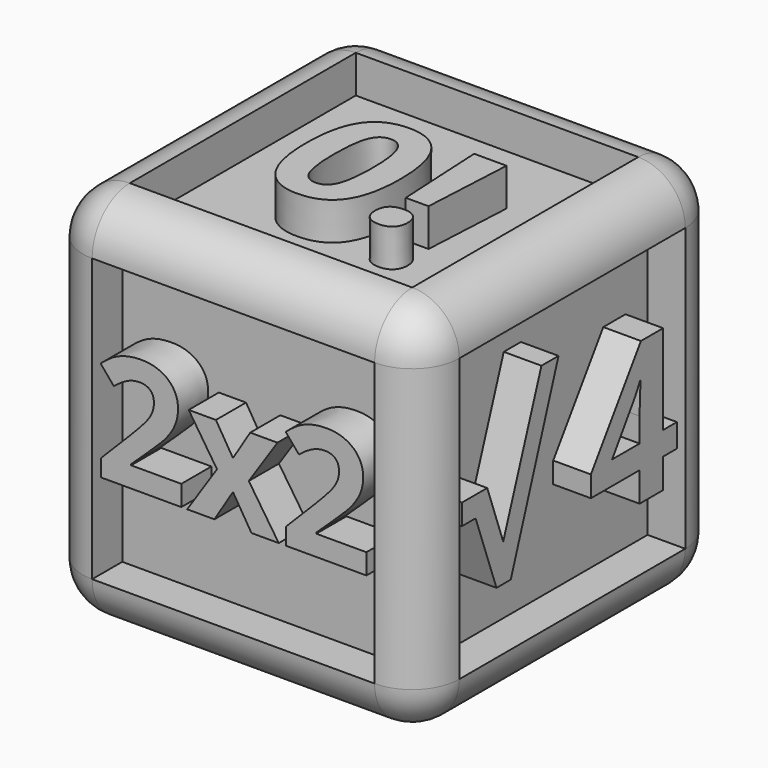
from build123d import *

# Parameters (mm, degrees)
F0_W          = 40
F0_H          = 40
F1_DEPTH      = 40
F2_R          = 5
F3_DEPTH      = 4
F4_DEPTH      = 4
F5_DEPTH      = 4
F6_DEPTH      = 4
F7_DEPTH      = 4
F8_DEPTH      = 4
F9_TEXT_SIZE  = 20.370244359
F10_DEPTH     = 4
F11_TEXT_SIZE = 21.2128028377
F12_DEPTH     = 4
F13_TEXT_SIZE = 18.89391852
F14_DEPTH     = 4
F15_TEXT_SIZE = 17.1153503298
F16_DEPTH     = 4
F17_TEXT_SIZE = 8.0331366888
F18_DEPTH     = 4
F19_TEXT_SIZE = 23.1590374525
F20_DEPTH     = 4


# Not quite as in the source:
# - Text() gives the source's letters only with a copy of the font that has no kerning and outlines rounded to 1/6400 em; it was checked with that copy


with BuildPart() as f1:
    # F0 (on Top) → F1 (new body)
    with BuildSketch(Plane.XY):
        Rectangle(F0_W, F0_H)
    extrude(amount=F1_DEPTH)

    # F2
    f2_edges = [f1.edges().sort_by_distance(p)[0] for p in [
        (0, -20, 40),
        (20, 0, 40),
        (0, 20, 40),
        (-20, 0, 40),
        (0, -20, 0),
        (20, 0, 0),
        (0, 20, 0),
        (-20, 0, 0),
        (-20, -20, 20),
        (20, -20, 20),
        (20, 20, 20),
        (-20, 20, 20),
    ]]
    fillet(f2_edges, radius=F2_R)

    # F3 (cut): a face of the model
    f3_faces = [f1.faces().sort_by_distance(p)[0] for p in [
        (0, 0, 40),
    ]]
    extrude(f3_faces, amount=-F3_DEPTH, mode=Mode.SUBTRACT)

    # F4 (cut): a face of the model
    f4_faces = [f1.faces().sort_by_distance(p)[0] for p in [
        (0, 20, 20),
    ]]
    extrude(f4_faces, amount=-F4_DEPTH, mode=Mode.SUBTRACT)

    # F5 (cut): a face of the model
    f5_faces = [f1.faces().sort_by_distance(p)[0] for p in [
        (20, 0, 20),
    ]]
    extrude(f5_faces, amount=-F5_DEPTH, mode=Mode.SUBTRACT)

    # F6 (cut): a face of the model
    f6_faces = [f1.faces().sort_by_distance(p)[0] for p in [
        (0, -20, 20),
    ]]
    extrude(f6_faces, amount=-F6_DEPTH, mode=Mode.SUBTRACT)

    # F7 (cut): a face of the model
    f7_faces = [f1.faces().sort_by_distance(p)[0] for p in [
        (-20, 0, 20),
    ]]
    extrude(f7_faces, amount=-F7_DEPTH, mode=Mode.SUBTRACT)

    # F8 (cut): a face of the model
    f8_faces = [f1.faces().sort_by_distance(p)[0] for p in [
        (0, 0, 0),
    ]]
    extrude(f8_faces, amount=-F8_DEPTH, mode=Mode.SUBTRACT)

    # F9 (on face) → F10 (join)
    with BuildSketch(Plane.XY.offset(36)):
        with Locations((-8.8264212281, -7.5825717722)):
            Text('0!', F9_TEXT_SIZE, font='Open Sans', font_style=FontStyle.BOLD, text_align=(TextAlign.LEFT, TextAlign.BOTTOM))
    extrude(amount=F10_DEPTH)

    # F11 (on face) → F12 (join)
    with BuildSketch(Plane.YZ.offset(16)):
        with Locations((-15.0464065373, 11.6780204698)):
            Text('√ 4', F11_TEXT_SIZE, font='Open Sans', font_style=FontStyle.BOLD, text_align=(TextAlign.LEFT, TextAlign.BOTTOM))
    extrude(amount=F12_DEPTH)

    # F13 (on face) → F14 (join)
    with BuildSketch(Plane(origin=(0, 16, 0), x_dir=(-1, 0, 0), z_dir=(0, 1, 0))):
        with Locations((-15, 14.4627944895)):
            Text('6/2', F13_TEXT_SIZE, font='Open Sans', font_style=FontStyle.BOLD, text_align=(TextAlign.LEFT, TextAlign.BOTTOM))
    extrude(amount=F14_DEPTH)

    # F15 (on face) → F16 (join)
    with BuildSketch(Plane.XZ.offset(16)):
        with Locations((-14.7576909291, 14.8219242724)):
            Text('2x2', F15_TEXT_SIZE, font='Open Sans', font_style=FontStyle.BOLD, text_align=(TextAlign.LEFT, TextAlign.BOTTOM))
    extrude(amount=F16_DEPTH)

    # F17 (on face) → F18 (join)
    with BuildSketch(Plane(origin=(-16, 0, 0), x_dir=(0, -1, 0), z_dir=(-1, 0, 0))):
        with Locations((-15, 18.1488376111)):
            Text('5 cos(0)', F17_TEXT_SIZE, font='Open Sans', font_style=FontStyle.BOLD, text_align=(TextAlign.LEFT, TextAlign.BOTTOM))
    extrude(amount=F18_DEPTH)

    # F19 (on face) → F20 (join)
    with BuildSketch(Plane(origin=(0, 0, 4), x_dir=(1, 0, 0), z_dir=(0, 0, -1))):
        with Locations((-10, -7.853056553)):
            Text('3!', F19_TEXT_SIZE, font='Open Sans', font_style=FontStyle.BOLD, text_align=(TextAlign.LEFT, TextAlign.BOTTOM))
    extrude(amount=F20_DEPTH)


solid = f1.part
